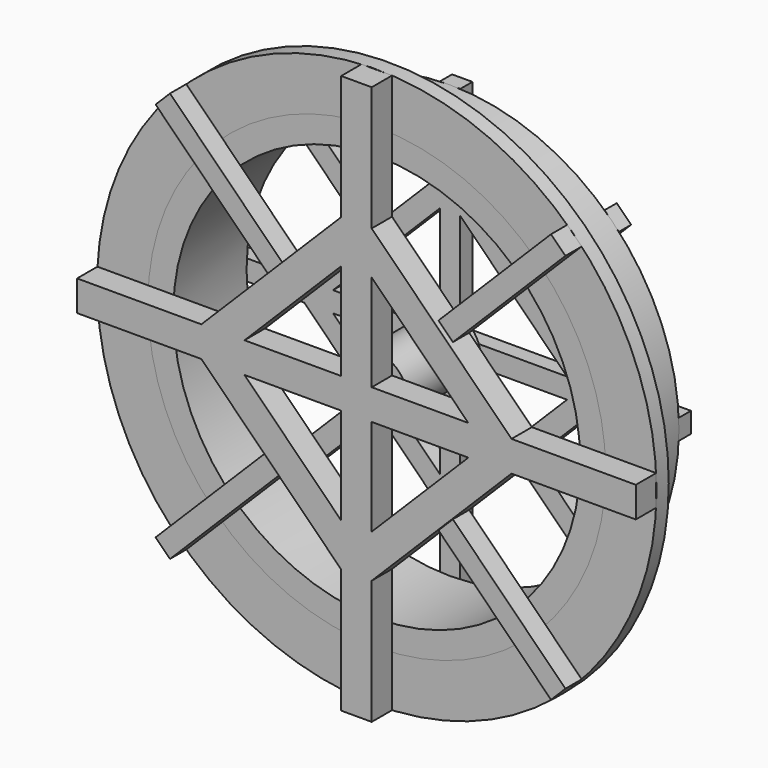
from build123d import *

# Parameters (mm, degrees)
F0_R      = 6
F1_DEPTH  = 18
F0_R_2    = 45
F0_R_3    = 40
F2_R      = 55
F2_R_2    = 45
F3_DEPTH  = 3
F4_W      = 6
F4_H      = 6
F5_DEPTH  = 5
F7_DEPTH  = 4
F9_DEPTH  = 1
F11_DEPTH = 2
F13_DEPTH = 2
F15_DEPTH = 2
F16_W     = 4
F16_H     = 4
F17_DEPTH = 3


with BuildPart() as f1:
    # F0 (on Front) → F1 (new body)
    with BuildSketch(Plane.XZ):
        Circle(F0_R)
    extrude(amount=F1_DEPTH)


with BuildPart() as f1b:
    # F0 (on Front) → F1, piece 2 (new body)
    with BuildSketch(Plane.XZ):
        Circle(F0_R_2)
        Circle(F0_R_3, mode=Mode.SUBTRACT)
    extrude(amount=F1_DEPTH)


with BuildPart() as f3:
    # F2 (on face) → F3 (new body)
    with BuildSketch(Plane.XZ.offset(18)):
        Circle(F2_R)
        Circle(F2_R_2, mode=Mode.SUBTRACT)
    extrude(amount=-F3_DEPTH)


with BuildPart() as f5:
    # F4 (on face) → F5 (new body)
    with BuildSketch(Plane.XZ.offset(18)):
        Rectangle(F4_W, F4_H)
        with BuildLine():
            Line((-54.918120871, 3), (-54.918120871, -3))
            Line((-54.918120871, -3), (-44.8998886413, -3))
            ThreePointArc((-44.8998886413, -3), (-45, 0), (-44.8998886413, 3))
            Line((-44.8998886413, 3), (-54.918120871, 3))
        make_face()
        Polygon((-25, 0), (-22, -3), (-3, -3), (-3, 3), (-22, 3), align=None)
        Polygon((3, -3), (-3, -3), (-3, -22), (0, -25), (3, -22), align=None)
        Polygon((3, 3), (3, -3), (22, -3), (25, 0), (22, 3), align=None)
        with BuildLine():
            Line((44.8998886413, -3), (54.918120871, -3))
            Line((54.918120871, -3), (54.918120871, 3))
            Line((54.918120871, 3), (44.8998886413, 3))
            ThreePointArc((44.8998886413, 3), (44.9749651965, 1.500834958), (45, 0))
            ThreePointArc((45, 0), (44.9749651965, -1.500834958), (44.8998886413, -3))
        make_face()
        with BuildLine():
            Line((3, 54.918120871), (-3, 54.918120871))
            Line((-3, 54.918120871), (-3, 44.8998886413))
            ThreePointArc((-3, 44.8998886413), (0, 45), (3, 44.8998886413))
            Line((3, 44.8998886413), (3, 54.918120871))
        make_face()
        with BuildLine():
            Line((-3, -44.8998886413), (-3, -54.918120871))
            Line((-3, -54.918120871), (3, -54.918120871))
            Line((3, -54.918120871), (3, -44.8998886413))
            ThreePointArc((3, -44.8998886413), (0, -45), (-3, -44.8998886413))
        make_face()
        Polygon((-3, 22), (-3, 3), (3, 3), (3, 22), (0, 25), align=None)
        with BuildLine():
            ThreePointArc((-44.8998886413, 3), (-45, 0), (-44.8998886413, -3))
            Line((-44.8998886413, -3), (-30.4852813742, -3))
            Line((-30.4852813742, -3), (-33.4852813742, 0))
            Line((-33.4852813742, 0), (-30.4852813742, 3))
            Line((-30.4852813742, 3), (-44.8998886413, 3))
        make_face()
        Polygon((-33.4852813742, 0), (-30.4852813742, -3), (-22, -3), (-25, 0), (-22, 3), (-30.4852813742, 3), align=None)
        Polygon((-3, 30.4852813742), (-30.4852813742, 3), (-22, 3), (-3, 22), align=None)
        Polygon((-22, -3), (-30.4852813742, -3), (-3, -30.4852813742), (-3, -22), align=None)
        Polygon((3, -22), (3, -30.4852813742), (30.4852813742, -3), (22, -3), align=None)
        Polygon((-3, -22), (-3, -30.4852813742), (0, -33.4852813742), (3, -30.4852813742), (3, -22), (0, -25), align=None)
        with BuildLine():
            Line((-3, -30.4852813742), (-3, -44.8998886413))
            ThreePointArc((-3, -44.8998886413), (0, -45), (3, -44.8998886413))
            Line((3, -44.8998886413), (3, -30.4852813742))
            Line((3, -30.4852813742), (0, -33.4852813742))
            Line((0, -33.4852813742), (-3, -30.4852813742))
        make_face()
        Polygon((30.4852813742, 3), (3, 30.4852813742), (3, 22), (22, 3), align=None)
        Polygon((22, -3), (30.4852813742, -3), (33.4852813742, 0), (30.4852813742, 3), (22, 3), (25, 0), align=None)
        Polygon((0, 33.4852813742), (-3, 30.4852813742), (-3, 22), (0, 25), (3, 22), (3, 30.4852813742), align=None)
        with BuildLine():
            ThreePointArc((3, 44.8998886413), (0, 45), (-3, 44.8998886413))
            Line((-3, 44.8998886413), (-3, 30.4852813742))
            Line((-3, 30.4852813742), (0, 33.4852813742))
            Line((0, 33.4852813742), (3, 30.4852813742))
            Line((3, 30.4852813742), (3, 44.8998886413))
        make_face()
        with BuildLine():
            Line((30.4852813742, -3), (44.8998886413, -3))
            ThreePointArc((44.8998886413, -3), (44.9749651965, -1.500834958), (45, 0))
            ThreePointArc((45, 0), (44.9749651965, 1.500834958), (44.8998886413, 3))
            Line((44.8998886413, 3), (30.4852813742, 3))
            Line((30.4852813742, 3), (33.4852813742, 0))
            Line((33.4852813742, 0), (30.4852813742, -3))
        make_face()
    extrude(amount=F5_DEPTH)


with BuildPart() as f7:
    # F6 (on face) → F7 (new body)
    with BuildSketch(Plane.XZ.offset(18)):
        Polygon((-40.279365048, 37.4509379232), (-15.5306277065, 12.7022005817), (-12.7022005817, 15.5306277065), (-37.4509379232, 40.279365048), align=None)
    extrude(amount=F7_DEPTH)

    # F8 (on face) → F9 (cut)
    with BuildSketch(Plane(origin=(0, -18, 0), x_dir=(-1, 0, 0), z_dir=(0, 1, 0))):
        Polygon((17.2983946594, 14.4699675347), (14.4699675347, 17.2983946594), (12.7022005817, 15.5306277065), (15.5306277065, 12.7022005817), align=None)
    extrude(amount=-F9_DEPTH, mode=Mode.SUBTRACT)


with BuildPart() as f7b:
    # F6 (on face) → F7, piece 2 (new body)
    with BuildSketch(Plane.XZ.offset(18)):
        Polygon((-15.5306277065, -12.7022005817), (-40.279365048, -37.4509379232), (-37.4509379232, -40.279365048), (-12.7022005817, -15.5306277065), align=None)
    extrude(amount=F7_DEPTH)

    # F10 (on face) → F11 (cut)
    with BuildSketch(Plane(origin=(0, -18, 0), x_dir=(-1, 0, 0), z_dir=(0, 1, 0))):
        Polygon((17.2983946594, -14.4699675347), (15.5306277065, -12.7022005817), (12.7022005817, -15.5306277065), (14.4699675347, -17.2983946594), align=None)
    extrude(amount=-F11_DEPTH, mode=Mode.SUBTRACT)


with BuildPart() as f7c:
    # F6 (on face) → F7, piece 3 (new body)
    with BuildSketch(Plane.XZ.offset(18)):
        Polygon((12.7022005817, -15.5306277065), (37.4509379232, -40.279365048), (40.279365048, -37.4509379232), (15.5306277065, -12.7022005817), align=None)
    extrude(amount=F7_DEPTH)

    # F12 (on face) → F13 (cut)
    with BuildSketch(Plane(origin=(0, -18, 0), x_dir=(-1, 0, 0), z_dir=(0, 1, 0))):
        Polygon((-14.8235209253, -17.65194805), (-12.7022005817, -15.5306277065), (-15.5306277065, -12.7022005817), (-17.65194805, -14.8235209253), align=None)
    extrude(amount=-F13_DEPTH, mode=Mode.SUBTRACT)


with BuildPart() as f7d:
    # F6 (on face) → F7, piece 4 (new body)
    with BuildSketch(Plane.XZ.offset(18)):
        Polygon((15.5306277065, 12.7022005817), (40.279365048, 37.4509379232), (37.4509379232, 40.279365048), (12.7022005817, 15.5306277065), align=None)
    extrude(amount=F7_DEPTH)

    # F14 (on face) → F15 (cut)
    with BuildSketch(Plane(origin=(0, -18, 0), x_dir=(-1, 0, 0), z_dir=(0, 1, 0))):
        Polygon((-15.5306277065, 12.7022005817), (-12.7022005817, 15.5306277065), (-14.8235209253, 17.65194805), (-17.65194805, 14.8235209253), align=None)
    extrude(amount=-F15_DEPTH, mode=Mode.SUBTRACT)


with BuildPart() as f17:
    # F16 (on face) → F17 (new body)
    with BuildSketch(Plane(origin=(0, 0, 0), x_dir=(-1, 0, 0), z_dir=(0, 1, 0))):
        with BuildLine():
            Line((-44.955533586, 2), (-44.955533586, -2))
            Line((-44.955533586, -2), (-39.9499687109, -2))
            ThreePointArc((-39.9499687109, -2), (-40, 0), (-39.9499687109, 2))
            Line((-39.9499687109, 2), (-44.955533586, 2))
        make_face()
        with BuildLine():
            ThreePointArc((-39.9499687109, 2), (-40, 0), (-39.9499687109, -2))
            Line((-39.9499687109, -2), (-28.6568542495, -2))
            Line((-28.6568542495, -2), (-30.6568542495, 0))
            Line((-30.6568542495, 0), (-28.6568542495, 2))
            Line((-28.6568542495, 2), (-39.9499687109, 2))
        make_face()
        with BuildLine():
            Line((-2, -39.9499687109), (-2, -44.955533586))
            Line((-2, -44.955533586), (2, -44.955533586))
            Line((2, -44.955533586), (2, -39.9499687109))
            ThreePointArc((2, -39.9499687109), (0, -40), (-2, -39.9499687109))
        make_face()
        Polygon((-30.6568542495, 0), (-28.6568542495, -2), (-23, -2), (-25, 0), (-23, 2), (-28.6568542495, 2), align=None)
        Polygon((-23, -2), (-28.6568542495, -2), (-16.7426406871, -13.9142135624), (-13.9142135624, -16.7426406871), (-2, -28.6568542495), (-2, -23), align=None)
        with BuildLine():
            ThreePointArc((-26.8346802213, -29.663107346), (-28.2842712475, -28.2842712475), (-29.663107346, -26.8346802213))
            Line((-29.663107346, -26.8346802213), (-33.1865494443, -30.3581223196))
            Line((-33.1865494443, -30.3581223196), (-30.3581223196, -33.1865494443))
            Line((-30.3581223196, -33.1865494443), (-26.8346802213, -29.663107346))
        make_face()
        with BuildLine():
            Line((-16.7426406871, -13.9142135624), (-29.663107346, -26.8346802213))
            ThreePointArc((-29.663107346, -26.8346802213), (-28.2842712475, -28.2842712475), (-26.8346802213, -29.663107346))
            Line((-26.8346802213, -29.663107346), (-13.9142135624, -16.7426406871))
            Line((-13.9142135624, -16.7426406871), (-16.7426406871, -13.9142135624))
        make_face()
        with BuildLine():
            Line((-30.3741490881, 33.2025762129), (-33.2025762129, 30.3741490881))
            Line((-33.2025762129, 30.3741490881), (-29.663107346, 26.8346802213))
            ThreePointArc((-29.663107346, 26.8346802213), (-28.2842712475, 28.2842712475), (-26.8346802213, 29.663107346))
            Line((-26.8346802213, 29.663107346), (-30.3741490881, 33.2025762129))
        make_face()
        with BuildLine():
            Line((-2, -28.6568542495), (-2, -39.9499687109))
            ThreePointArc((-2, -39.9499687109), (0, -40), (2, -39.9499687109))
            Line((2, -39.9499687109), (2, -28.6568542495))
            Line((2, -28.6568542495), (0, -30.6568542495))
            Line((0, -30.6568542495), (-2, -28.6568542495))
        make_face()
        Polygon((-25, 0), (-23, -2), (-2, -2), (-2, 2), (-23, 2), align=None)
        Polygon((-16.7426406871, 13.9142135624), (-28.6568542495, 2), (-23, 2), (-2, 23), (-2, 28.6568542495), (-13.9142135624, 16.7426406871), align=None)
        with BuildLine():
            ThreePointArc((-26.8346802213, 29.663107346), (-28.2842712475, 28.2842712475), (-29.663107346, 26.8346802213))
            Line((-29.663107346, 26.8346802213), (-16.7426406871, 13.9142135624))
            Line((-16.7426406871, 13.9142135624), (-13.9142135624, 16.7426406871))
            Line((-13.9142135624, 16.7426406871), (-26.8346802213, 29.663107346))
        make_face()
        with BuildLine():
            Line((39.9499687109, -2), (44.955533586, -2))
            Line((44.955533586, -2), (44.955533586, 2))
            Line((44.955533586, 2), (39.9499687109, 2))
            ThreePointArc((39.9499687109, 2), (39.9874902215, 1.0003128423), (40, 0))
            ThreePointArc((40, 0), (39.9874902215, -1.0003128423), (39.9499687109, -2))
        make_face()
        Polygon((-2, -23), (-2, -28.6568542495), (0, -30.6568542495), (2, -28.6568542495), (2, -23), (0, -25), align=None)
        Rectangle(F16_W, F16_H)
        Polygon((2, -2), (-2, -2), (-2, -23), (0, -25), (2, -23), align=None)
        with BuildLine():
            Line((2, 44.955533586), (-2, 44.955533586))
            Line((-2, 44.955533586), (-2, 39.9499687109))
            ThreePointArc((-2, 39.9499687109), (0, 40), (2, 39.9499687109))
            Line((2, 39.9499687109), (2, 44.955533586))
        make_face()
        Polygon((2, -23), (2, -28.6568542495), (13.9302403309, -16.7266139185), (16.7586674557, -13.8981867938), (28.6568542495, -2), (23, -2), align=None)
        with BuildLine():
            ThreePointArc((29.6783272148, -26.8178465529), (28.3003135351, -28.2682198558), (26.8515047742, -29.6478783618))
            Line((26.8515047742, -29.6478783618), (30.3741490881, -33.1705226757))
            Line((30.3741490881, -33.1705226757), (33.2025762129, -30.342095551))
            Line((33.2025762129, -30.342095551), (29.6783272148, -26.8178465529))
        make_face()
        with BuildLine():
            Line((13.9302403309, -16.7266139185), (26.8515047742, -29.6478783618))
            ThreePointArc((26.8515047742, -29.6478783618), (28.3003135351, -28.2682198558), (29.6783272148, -26.8178465529))
            Line((29.6783272148, -26.8178465529), (16.7586674557, -13.8981867938))
            Line((16.7586674557, -13.8981867938), (13.9302403309, -16.7266139185))
        make_face()
        with BuildLine():
            Line((28.6568542495, -2), (39.9499687109, -2))
            ThreePointArc((39.9499687109, -2), (39.9874902215, -1.0003128423), (40, 0))
            ThreePointArc((40, 0), (39.9874902215, 1.0003128423), (39.9499687109, 2))
            Line((39.9499687109, 2), (28.6568542495, 2))
            Line((28.6568542495, 2), (30.6568542495, 0))
            Line((30.6568542495, 0), (28.6568542495, -2))
        make_face()
        Polygon((2, 2), (2, -2), (23, -2), (25, 0), (23, 2), align=None)
        Polygon((-2, 23), (-2, 2), (2, 2), (2, 23), (0, 25), align=None)
        Polygon((-2, 28.6568542495), (-2, 23), (0, 25), (2, 23), (2, 28.6568542495), (0, 30.6568542495), align=None)
        with BuildLine():
            ThreePointArc((2, 39.9499687109), (0, 40), (-2, 39.9499687109))
            Line((-2, 39.9499687109), (-2, 28.6568542495))
            Line((-2, 28.6568542495), (0, 30.6568542495))
            Line((0, 30.6568542495), (2, 28.6568542495))
            Line((2, 28.6568542495), (2, 39.9499687109))
        make_face()
        Polygon((23, -2), (28.6568542495, -2), (30.6568542495, 0), (28.6568542495, 2), (23, 2), (25, 0), align=None)
        with BuildLine():
            ThreePointArc((30.357405266, 33.2178859279), (30.3657781419, 33.2102321256), (30.3741490881, 33.2025762129))
            Line((30.3741490881, 33.2025762129), (30.3581223196, 33.2186029814))
            Line((30.3581223196, 33.2186029814), (30.357405266, 33.2178859279))
        make_face()
        with BuildLine():
            Line((33.1865494443, 30.3901758567), (30.3741490881, 33.2025762129))
            ThreePointArc((30.3741490881, 33.2025762129), (30.3657781419, 33.2102321256), (30.357405266, 33.2178859279))
            Line((30.357405266, 33.2178859279), (26.8178465529, 29.6783272148))
            ThreePointArc((26.8178465529, 29.6783272148), (28.2682198558, 28.3003135351), (29.6478783618, 26.8515047742))
            Line((29.6478783618, 26.8515047742), (33.1865494443, 30.3901758567))
        make_face()
        Polygon((23, 2), (28.6568542495, 2), (16.7266139185, 13.9302403309), (13.8981867938, 16.7586674557), (2, 28.6568542495), (2, 23), align=None)
        with BuildLine():
            Line((16.7266139185, 13.9302403309), (29.6478783618, 26.8515047742))
            ThreePointArc((29.6478783618, 26.8515047742), (28.2682198558, 28.3003135351), (26.8178465529, 29.6783272148))
            Line((26.8178465529, 29.6783272148), (13.8981867938, 16.7586674557))
            Line((13.8981867938, 16.7586674557), (16.7266139185, 13.9302403309))
        make_face()
    extrude(amount=F17_DEPTH)


solid = Compound([f1.part, f1b.part, f3.part, f5.part, f7.part, f7b.part, f7c.part, f7d.part, f17.part])
